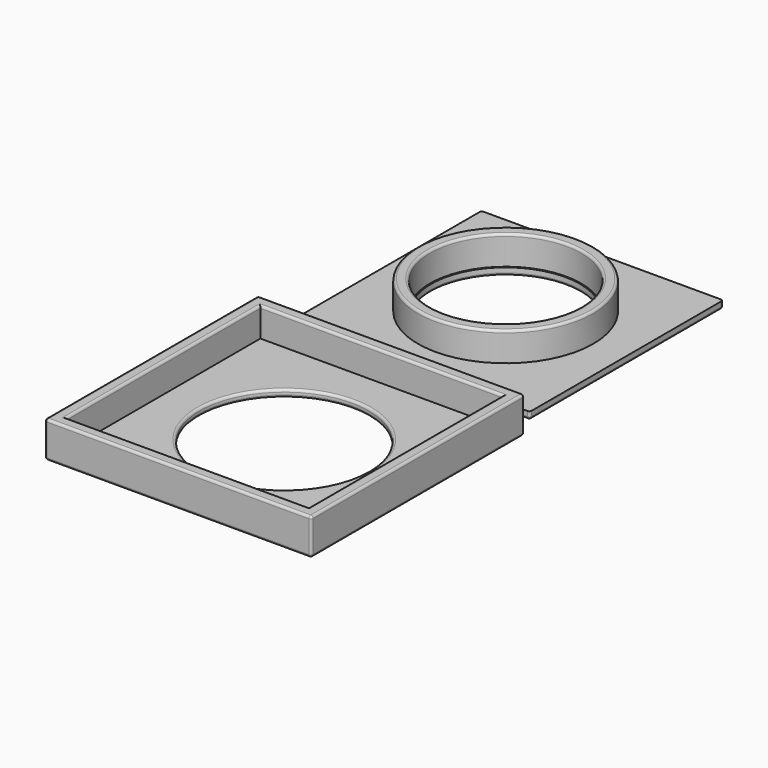
from build123d import *

# Parameters (mm, degrees)
F0_R     = 36.3
F0_R_2   = 31.3
F1_DEPTH = 15
F0_W     = 110.2
F0_H     = 110.2
F0_W_2   = 100.2
F0_H_2   = 100.2
F0_W_3   = 100
F0_H_3   = 100
F0_R_3   = 30.8
F2_DEPTH = 3
F0_R_4   = 35
F3_R     = 1
F3_2_R   = 1


# Not quite as in the source:
# - a feature names something its author has since deleted; it is built from what else it names


with BuildPart() as f1:
    # F0 (on Top) → F1 (new body)
    with BuildSketch(Plane.XY):
        with Locations((50, 50)):
            Circle(F0_R)
        with Locations((50, 50)):
            Circle(F0_R_2, mode=Mode.SUBTRACT)
    extrude(amount=F1_DEPTH)

    # F0 (on Top) → F2 (join)
    with BuildSketch(Plane.XY):
        with Locations((50, 50)):
            Rectangle(F0_W_3, F0_H_3)
        with Locations((50, 50)):
            Circle(F0_R, mode=Mode.SUBTRACT)
        with Locations((50, 50)):
            Circle(F0_R_2)
        with Locations((50, 50)):
            Circle(F0_R_3, mode=Mode.SUBTRACT)
    extrude(amount=F2_DEPTH)

    # F3
    f3_edges = [f1.edges().sort_by_distance(p)[0] for p in [
        (18.7, 50, 15),
        (13.7, 50, 15),
        (50, 0, 0),
        (100, 50, 0),
        (50, 100, 0),
        (0, 50, 0),
        (19.2, 50, 0),
        (100, 100, 1.5),
        (0, 100, 1.5),
        (0, 0, 1.5),
        (100, 0, 1.5),
    ]]
    fillet(f3_edges, radius=F3_R)


with BuildPart() as f1b:
    # F0 (on Top) → F1, piece 2 (new body)
    with BuildSketch(Plane.XY):
        with Locations((50.1000001118, -64.4040923819)):
            Rectangle(F0_W, F0_H)
        with Locations((50.1, -64.4040924937)):
            Rectangle(F0_W_2, F0_H_2, mode=Mode.SUBTRACT)
    extrude(amount=F1_DEPTH)

    # F0 (on Top) → F2, piece 2 (join)
    with BuildSketch(Plane.XY):
        with Locations((50.1, -64.4040924937)):
            Rectangle(F0_W_2, F0_H_2)
        with Locations((50.1, -64.6040926054)):
            Circle(F0_R_4, mode=Mode.SUBTRACT)
    extrude(amount=F2_DEPTH)

    # F3#2
    f3_2_edges = [f1b.edges().sort_by_distance(p)[0] for p in [
        (105.2, -64.404092, 15),
        (50.1, -9.304092, 15),
        (-5, -64.404092, 15),
        (50.1, -119.504092, 15),
        (-5, -119.504092, 7.5),
        (105.2, -119.504092, 7.5),
        (105.2, -9.304092, 7.5),
        (-5, -9.304092, 7.5),
        (50.1, -9.304092, 0),
        (105.2, -64.404092, 0),
        (15.1, -64.604093, 0),
        (-5, -64.404092, 0),
        (50.1, -119.504092, 0),
        (15.1, -64.604093, 3),
        (0, -64.404092, 15),
        (50.1, -14.304092, 15),
        (100.2, -64.404092, 15),
        (50.1, -114.504092, 15),
    ]]
    fillet(f3_2_edges, radius=F3_2_R)


solid = Compound([f1.part, f1b.part])
